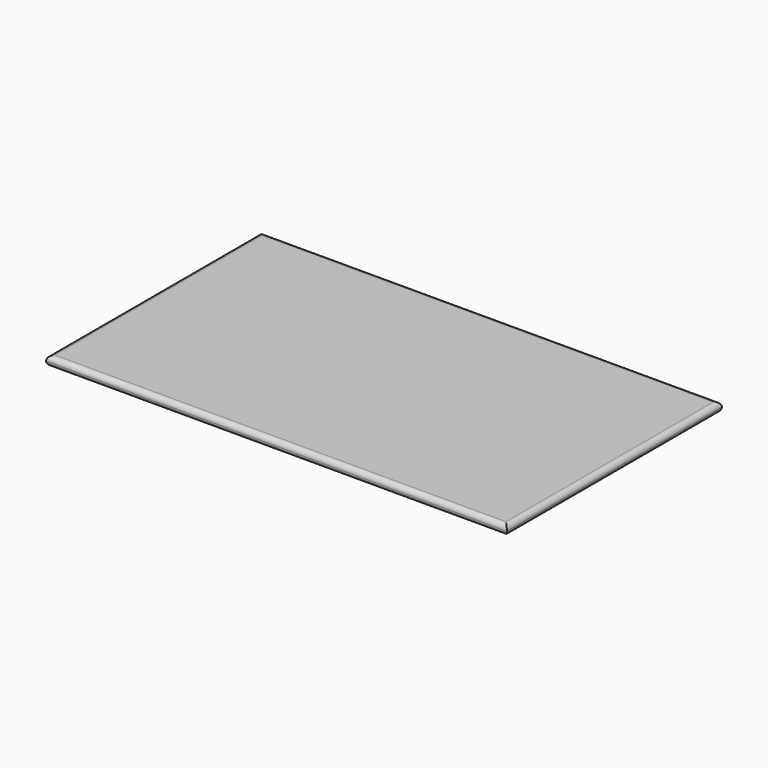
from build123d import *

# Parameters (mm, degrees)
F0_W     = 1219.2
F0_H     = 711.2
F1_DEPTH = 25.4
F2_R     = 12.69999


# Not quite as in the source:
# - a fillet or chamfer is up to 0.001 mm smaller than in the source, because OpenCascade refuses the exact size


with BuildPart() as f1:
    # F0 (on Top) → F1 (new body)
    with BuildSketch(Plane.XY):
        Rectangle(F0_W, F0_H)
    extrude(amount=F1_DEPTH)

    # F2 (radius 12.7 in the source; OpenCascade refuses exactly that, so slightly less here)
    f2_edges = [f1.edges().sort_by_distance(p)[0] for p in [
        (609.6, 0, 25.4),
        (0, 355.6, 25.4),
        (-609.6, 0, 25.4),
        (0, -355.6, 25.4),
        (609.6, 0, 0),
        (0, 355.6, 0),
        (-609.6, 0, 0),
        (0, -355.6, 0),
    ]]
    fillet(f2_edges, radius=F2_R)


solid = f1.part
